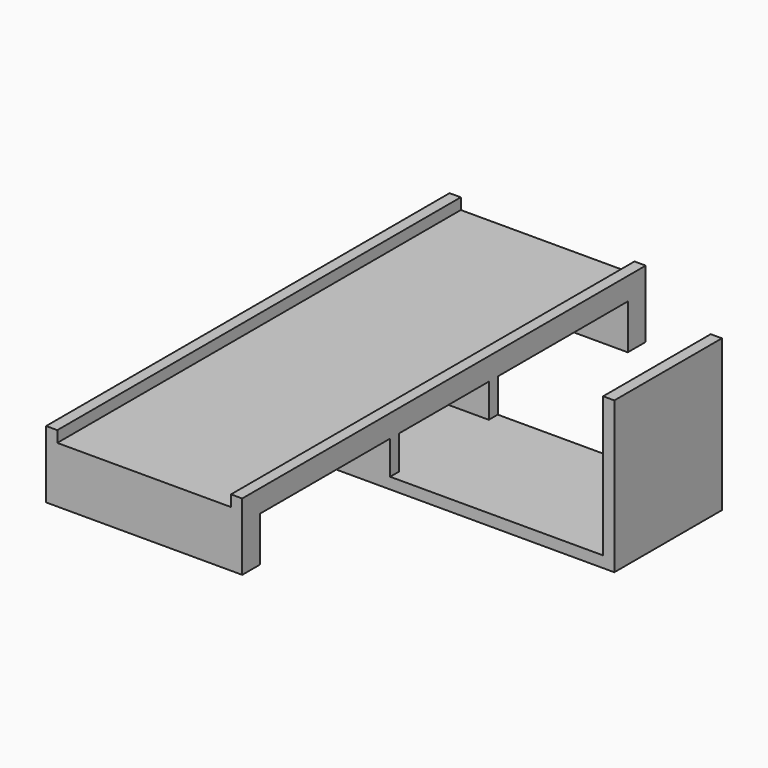
from build123d import *

# Parameters (mm, degrees)
F0_W      = 350
F0_H      = 900
F1_DEPTH  = 20
F2_W      = 100
F2_H      = 20
F3_DEPTH  = 175
F4_W      = 350
F4_H      = 40
F5_DEPTH  = 80
F6_W      = 20
F6_H      = 900
F7_DEPTH  = 20
F8_W      = 240
F8_H      = 20
F9_DEPTH  = 400
F10_W     = 20
F10_H     = 240
F11_DEPTH = 250
F12_R     = 5
F13_DEPTH = 20.001


# Not quite as in the source:
# - a pattern or mirror of a feature is missing from the dataset's text; its kind, count and spacing are read off the source's solid


with BuildPart() as f1:
    # F0 (on Top) → F1 (new body)
    with BuildSketch(Plane.XY):
        Rectangle(F0_W, F0_H)
    extrude(amount=F1_DEPTH)

    # F2 (on Right) → F3 (join, symmetric)
    with BuildSketch(Plane.YZ):
        Polygon((-100, 0), (-120, 0), (-120, -80), (-100, -80), (-100, -60), align=None)
        with Locations((-50, -70)):
            Rectangle(F2_W, F2_H)
    f3 = extrude(amount=F3_DEPTH, both=True)

    # F3_copies: F3 across plane
    add(f3.mirror(Plane.ZX))

    # F4 (on face) → F5 (join)
    with BuildSketch(Plane(origin=(0, 0, 0), x_dir=(1, 0, 0), z_dir=(0, 0, -1))):
        with Locations((0, 430)):
            Rectangle(F4_W, F4_H)
    f5 = extrude(amount=F5_DEPTH)

    # F5_copies: F5 across plane
    add(f5.mirror(Plane.ZX))

    # F6 (on face) → F7 (join)
    with BuildSketch(Plane.XY.offset(20)):
        with Locations((-165, 0)):
            Rectangle(F6_W, F6_H)
        with Locations((165, 0)):
            Rectangle(F6_W, F6_H)
    extrude(amount=F7_DEPTH)

    # F8 (on face) → F9 (join)
    with BuildSketch(Plane.YZ.offset(175)):
        with Locations((0, -70)):
            Rectangle(F8_W, F8_H)
    extrude(amount=F9_DEPTH)

    # F10 (on face) → F11 (join)
    with BuildSketch(Plane.XY.offset(-60)):
        with Locations((565, 0)):
            Rectangle(F10_W, F10_H)
    extrude(amount=F11_DEPTH)

    # F12 (on face) → F13 (cut, through all)
    with BuildSketch(Plane.XY.offset(-60)):
        with Locations((525, 90)):
            Circle(F12_R)
        with Locations((485, 0)):
            Circle(F12_R)
    extrude(amount=-F13_DEPTH, mode=Mode.SUBTRACT)


solid = f1.part
